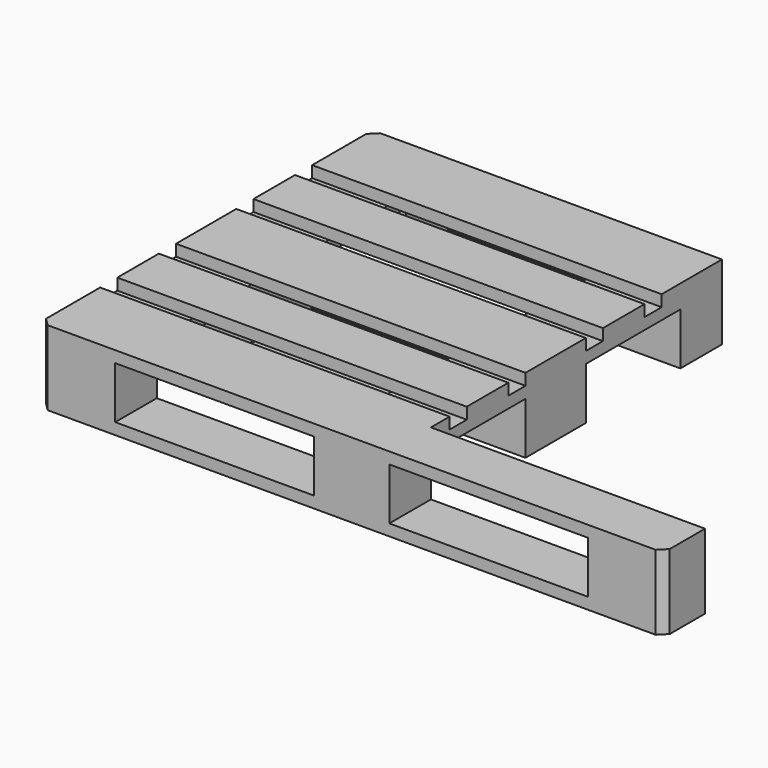
from build123d import *

# Parameters (mm, degrees)
F0_W      = 1200
F0_H      = 145
F1_DEPTH  = 22
F0_H_2    = 100
F2_W      = 145
F2_H      = 655
F2_H_2    = 145
F3_DEPTH  = 22
F4_W      = 145
F4_H      = 100
F6_DEPTH  = 78
F4_H_2    = 145
F5_W      = 145
F5_H      = 145
F5_H_2    = 100
F7_W      = 145
F7_H      = 100
F7_W_2    = 1055
F8_DEPTH  = 22
F7_W_3    = 1200
F7_H_2    = 145
F10_SIZE  = 15
F11_W     = 527.5
F11_H     = 145
F12_DEPTH = 211


# Not quite as in the source:
# - a feature names something its author has since deleted; it is built from what else it names


with BuildPart() as f1:
    # F0 (on Top) → F1 (new body)
    with BuildSketch(Plane.XY):
        with Locations((0, 327.5)):
            Rectangle(F0_W, F0_H)
    extrude(amount=-F1_DEPTH)


with BuildPart() as f1b:
    # F0 (on Top) → F1, piece 2 (new body)
    with BuildSketch(Plane.XY):
        with Locations((0, 163.75)):
            Rectangle(F0_W, F0_H_2)
    extrude(amount=-F1_DEPTH)


with BuildPart() as f1c:
    # F0 (on Top) → F1, piece 3 (new body)
    with BuildSketch(Plane.XY):
        Rectangle(F0_W, F0_H)
    extrude(amount=-F1_DEPTH)


with BuildPart() as f1d:
    # F0 (on Top) → F1, piece 4 (new body)
    with BuildSketch(Plane.XY):
        with Locations((0, -163.75)):
            Rectangle(F0_W, F0_H_2)
    extrude(amount=-F1_DEPTH)


with BuildPart() as f1e:
    # F0 (on Top) → F1, piece 5 (new body)
    with BuildSketch(Plane.XY):
        with Locations((0, -327.5)):
            Rectangle(F0_W, F0_H)
    extrude(amount=-F1_DEPTH)


with BuildPart() as f3:
    # F2 (on face) → F3 (new body)
    with BuildSketch(Plane(origin=(0, 0, -22), x_dir=(1, 0, 0), z_dir=(0, 0, -1))):
        with Locations((-527.5, -72.5)):
            Rectangle(F2_W, F2_H)
        with Locations((-527.5, 327.5)):
            Rectangle(F2_W, F2_H_2)
    extrude(amount=F3_DEPTH)


with BuildPart() as f3b:
    # F2 (on face) → F3, piece 2 (new body)
    with BuildSketch(Plane(origin=(0, 0, -22), x_dir=(1, 0, 0), z_dir=(0, 0, -1))):
        with Locations((0, 327.5)):
            Rectangle(F2_W, F2_H_2)
        with Locations((0, -72.5)):
            Rectangle(F2_W, F2_H)
    extrude(amount=F3_DEPTH)


with BuildPart() as f3c:
    # F2 (on face) → F3, piece 3 (new body)
    with BuildSketch(Plane(origin=(0, 0, -22), x_dir=(1, 0, 0), z_dir=(0, 0, -1))):
        with Locations((527.5, 327.5)):
            Rectangle(F2_W, F2_H_2)
        with Locations((527.5, -72.5)):
            Rectangle(F2_W, F2_H)
    extrude(amount=F3_DEPTH)


with BuildPart() as f6:
    # F4 (on face) → F6 (new body)
    with BuildSketch(Plane(origin=(0, 0, -44), x_dir=(1, 0, 0), z_dir=(0, 0, -1))):
        with Locations((-527.5, -350)):
            Rectangle(F4_W, F4_H)
    extrude(amount=F6_DEPTH)


with BuildPart() as f6b:
    # F4 (on face) → F6, piece 2 (new body)
    with BuildSketch(Plane(origin=(0, 0, -44), x_dir=(1, 0, 0), z_dir=(0, 0, -1))):
        with Locations((-527.5, 350)):
            Rectangle(F4_W, F4_H)
    extrude(amount=F6_DEPTH)


with BuildPart() as f6c:
    # F4 (on face) → F6, piece 3 (new body)
    with BuildSketch(Plane(origin=(0, 0, -44), x_dir=(1, 0, 0), z_dir=(0, 0, -1))):
        with Locations((527.5, -350)):
            Rectangle(F4_W, F4_H)
    extrude(amount=F6_DEPTH)


with BuildPart() as f6d:
    # F4 (on face) → F6, piece 4 (new body)
    with BuildSketch(Plane(origin=(0, 0, -44), x_dir=(1, 0, 0), z_dir=(0, 0, -1))):
        with Locations((527.5, 0)):
            Rectangle(F4_W, F4_H_2)
    extrude(amount=F6_DEPTH)


with BuildPart() as f6e:
    # F4 (on face) → F6, piece 5 (new body)
    with BuildSketch(Plane(origin=(0, 0, -44), x_dir=(1, 0, 0), z_dir=(0, 0, -1))):
        with Locations((527.5, 350)):
            Rectangle(F4_W, F4_H)
    extrude(amount=F6_DEPTH)


with BuildPart() as f6f:
    # F4 (on face) → F6, piece 6 (new body)
    with BuildSketch(Plane(origin=(0, 0, -44), x_dir=(1, 0, 0), z_dir=(0, 0, -1))):
        with Locations((-527.5, 0)):
            Rectangle(F4_W, F4_H_2)
    extrude(amount=F6_DEPTH)


with BuildPart() as f6g:
    # F5 (on face) → F6, piece 7 (new body)
    with BuildSketch(Plane(origin=(0, 0, -44), x_dir=(1, 0, 0), z_dir=(0, 0, -1))):
        Rectangle(F5_W, F5_H)
    extrude(amount=F6_DEPTH)


with BuildPart() as f6h:
    # F5 (on face) → F6, piece 8 (new body)
    with BuildSketch(Plane(origin=(0, 0, -44), x_dir=(1, 0, 0), z_dir=(0, 0, -1))):
        with Locations((0, 350)):
            Rectangle(F5_W, F5_H_2)
    extrude(amount=F6_DEPTH)


with BuildPart() as f6i:
    # F5 (on face) → F6, piece 9 (new body)
    with BuildSketch(Plane(origin=(0, 0, -44), x_dir=(1, 0, 0), z_dir=(0, 0, -1))):
        with Locations((0, -350)):
            Rectangle(F5_W, F5_H_2)
    extrude(amount=F6_DEPTH)


with BuildPart() as f8:
    # F7 (on face) → F8 (new body)
    with BuildSketch(Plane(origin=(0, 0, -122), x_dir=(1, 0, 0), z_dir=(0, 0, -1))):
        with Locations((-527.5, -350)):
            Rectangle(F7_W, F7_H)
        with Locations((72.5, -350)):
            Rectangle(F7_W_2, F7_H)
    extrude(amount=F8_DEPTH)


with BuildPart() as f8b:
    # F7 (on face) → F8, piece 2 (new body)
    with BuildSketch(Plane(origin=(0, 0, -122), x_dir=(1, 0, 0), z_dir=(0, 0, -1))):
        Rectangle(F7_W_3, F7_H_2)
    extrude(amount=F8_DEPTH)


with BuildPart() as f8c:
    # F7 (on face) → F8, piece 3 (new body)
    with BuildSketch(Plane(origin=(0, 0, -122), x_dir=(1, 0, 0), z_dir=(0, 0, -1))):
        with Locations((0, 350)):
            Rectangle(F7_W_3, F7_H)
    extrude(amount=F8_DEPTH)


with BuildPart() as f3c_1:
    add(f3c.part)

    # F9: union F3b, F3, F1, F1b, F1e, F1d, F1c, F6, F6b, F6d, F6f, F8b, F8c, F6e, F6c, F8, F6i, F6g, F6h
    add(f3b.part)
    add(f3.part)
    add(f1.part)
    add(f1b.part)
    add(f1e.part)
    add(f1d.part)
    add(f1c.part)
    add(f6.part)
    add(f6b.part)
    add(f6d.part)
    add(f6f.part)
    add(f8b.part)
    add(f8c.part)
    add(f6e.part)
    add(f6c.part)
    add(f8.part)
    add(f6i.part)
    add(f6g.part)
    add(f6h.part)

    # F10
    f10_edges = [f3c_1.edges().sort_by_distance(p)[0] for p in [
        (-600, -400, -72),
        (600, -400, -72),
        (600, 400, -72),
        (-600, 400, -72),
    ]]
    chamfer(f10_edges, length=F10_SIZE)

    # F11 (on face) → F12 (cut)
    with BuildSketch(Plane(origin=(0, 0, -144), x_dir=(1, 0, 0), z_dir=(0, 0, -1))):
        with Locations((336.25, 0)):
            Rectangle(F11_W, F11_H)
        Polygon((672.5, -500), (672.5, 300), (72.5, 300), (72.5, 72.5), (600, 72.5), (600, -72.5), (72.5, -72.5), (72.5, -500), align=None)
    extrude(amount=-F12_DEPTH, mode=Mode.SUBTRACT)


solid = f3c_1.part
